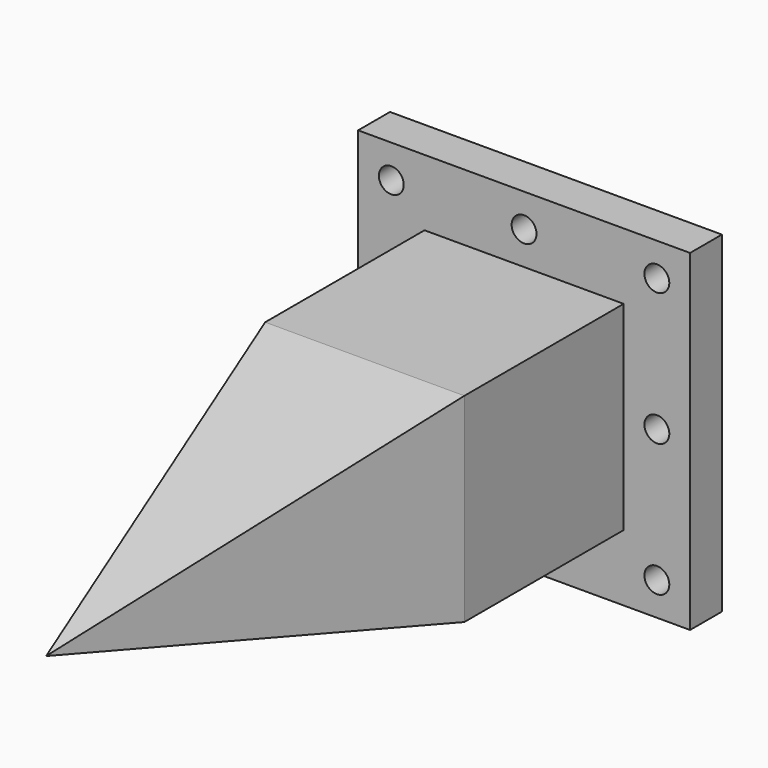
from build123d import *

# Parameters (mm, degrees)
F0_W     = 63.5
F0_H     = 63.5
F1_DEPTH = 7.62
F3_DEPTH = 114.3
F4_SIZE2 = 19.04999
F4_SIZE  = 76.19999
F5_R     = 2.38125
F7_DEPTH = 25.4
F9_DEPTH = 25.4


# Not quite as in the source:
# - a fillet or chamfer is up to 0.001 mm smaller than in the source, because OpenCascade refuses the exact size


with BuildPart() as f1:
    # F0 (on Front) → F1 (new body)
    with BuildSketch(Plane.XZ):
        with Locations((31.75, -31.75)):
            Rectangle(F0_W, F0_H)
    extrude(amount=F1_DEPTH)

    # F2 (on face) → F3 (join)
    with BuildSketch(Plane.XZ.offset(7.62)):
        Polygon((50.8, -12.7), (31.75, -12.7), (12.7, -12.7), (12.7, -50.8), (50.8, -50.8), align=None)
    extrude(amount=F3_DEPTH)

    # F4 (size 76.2 and 19.05 in the source; OpenCascade refuses exactly that, so slightly less here)
    f4_edges = [f1.edges().sort_by_distance(p)[0] for p in [
        (31.75, -121.92, -12.7),
        (12.7, -121.92, -31.75),
        (31.75, -121.92, -50.8),
        (50.8, -121.92, -31.75),
    ]]
    chamfer(f4_edges, length=F4_SIZE, length2=F4_SIZE2)

    # F5 (on face) → F7 (cut)
    with BuildSketch(Plane.XZ.offset(7.62)):
        with Locations((6.35, -6.35)):
            Circle(F5_R)
    extrude(amount=-F7_DEPTH, mode=Mode.SUBTRACT)

    # F5 (on face) → F9 (cut)
    with BuildSketch(Plane.XZ.offset(7.62)):
        with Locations((6.35, -31.75)):
            Circle(F5_R)
        with Locations((6.35, -57.15)):
            Circle(F5_R)
        with Locations((31.75, -57.15)):
            Circle(F5_R)
        with Locations((57.15, -57.15)):
            Circle(F5_R)
        with Locations((57.15, -31.75)):
            Circle(F5_R)
        with Locations((57.15, -6.35)):
            Circle(F5_R)
        with Locations((31.75, -6.35)):
            Circle(F5_R)
    extrude(amount=-F9_DEPTH, mode=Mode.SUBTRACT)


solid = f1.part
